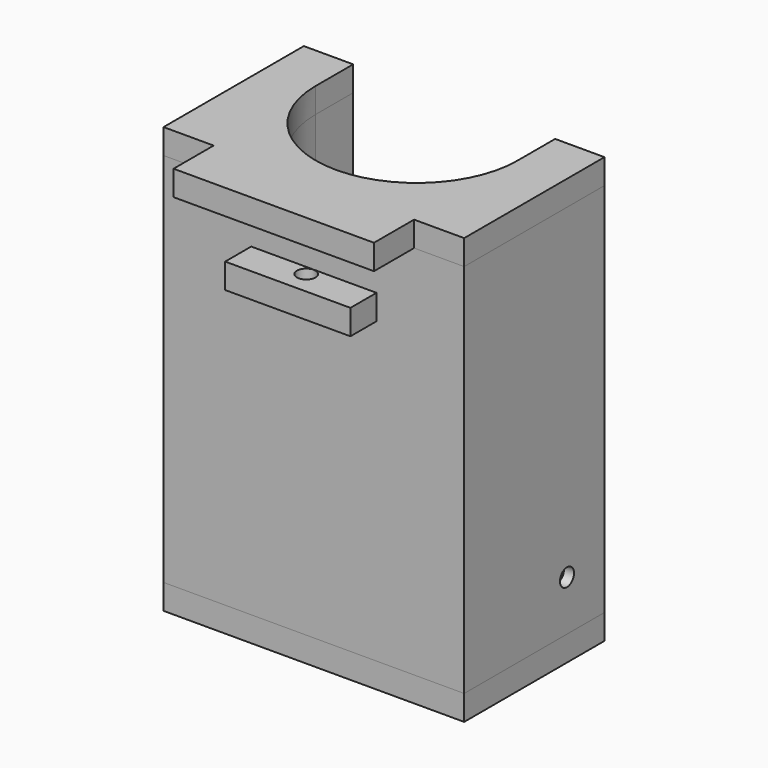
from build123d import *

# Parameters (mm, degrees)
F1_DEPTH  = 5
F3_DEPTH  = 2.1
F5_DEPTH  = 8.2
F7_DEPTH  = 60
F10_DEPTH = 5
F12_W     = 25
F12_H     = 6.5
F12_R     = 1.85
F13_DEPTH = 5
F15_R     = 1.75
F16_DEPTH = 3
F17_R     = 1.75
F18_DEPTH = 10
F20_W     = 3
F20_H     = 6.2998386914
F21_DEPTH = 25


# Not quite as in the source:
# - a pattern or mirror of a feature is missing from the dataset's text; its kind, count and spacing are read off the source's solid
# - a feature names something its author has since deleted; it is built from what else it names


with BuildPart() as f1:
    # F0 (on Top) → F1 (new body)
    with BuildSketch(Plane.XY):
        with BuildLine():
            Line((-20.15, 24), (-30, 24))
            Line((-30, 24), (-30, -11))
            Line((-30, -11), (-12.5, -11))
            Line((-12.5, -11), (30, -11))
            Line((30, -11), (30, 24))
            Line((30, 24), (20.15, 24))
            Line((20.15, 24), (20.15, 14.65))
            ThreePointArc((20.15, 14.65), (0, -5.5), (-20.15, 14.65))
            Line((-20.15, 14.65), (-20.15, 24))
        make_face()
    extrude(amount=F1_DEPTH)

    # F2 (on face) → F3 (join)
    with BuildSketch(Plane.XY.offset(5)):
        with BuildLine():
            Line((-20.15, 24), (-30, 24))
            Line((-30, 24), (-30, -11))
            Line((-30, -11), (30, -11))
            Line((30, -11), (30, 24))
            Line((30, 24), (20.15, 24))
            Line((20.15, 24), (20.15, 14.65))
            ThreePointArc((20.15, 14.65), (0, -5.5), (-20.15, 14.65))
            Line((-20.15, 14.65), (-20.15, 24))
        make_face()
    extrude(amount=F3_DEPTH)

    # F4 (on face) → F5 (join)
    with BuildSketch(Plane.XY.offset(7.1)):
        with BuildLine():
            Line((-22.6, 24), (-30, 24))
            Line((-30, 24), (-30, -11))
            Line((-30, -11), (30, -11))
            Line((30, -11), (30, 24))
            Line((30, 24), (22.6, 24))
            Line((22.6, 24), (22.6, 14.65))
            ThreePointArc((22.6, 14.65), (0, -7.95), (-22.6, 14.65))
            Line((-22.6, 14.65), (-22.6, 24))
        make_face()
    extrude(amount=F5_DEPTH)

    # F6 (on face) → F7 (join)
    with BuildSketch(Plane.XY.offset(15.3)):
        with BuildLine():
            Line((-20.15, 24), (-30, 24))
            Line((-30, 24), (-30, -11))
            Line((-30, -11), (30, -11))
            Line((30, -11), (30, 24))
            Line((30, 24), (20.15, 24))
            Line((20.15, 24), (20.15, 14.65))
            ThreePointArc((20.15, 14.65), (0, -5.5), (-20.15, 14.65))
            Line((-20.15, 14.65), (-20.15, 24))
        make_face()
    extrude(amount=F7_DEPTH)

    # F12 (on offset) → F13 (join)
    with BuildSketch(Plane.XY.offset(64.7)):
        with Locations((0, -14.25)):
            Rectangle(F12_W, F12_H)
        with Locations((0, -12.9)):
            Circle(F12_R, mode=Mode.SUBTRACT)
    extrude(amount=-F13_DEPTH)

    # F15 (on offset) → F16 (cut)
    with BuildSketch(Plane.YZ.offset(25)):
        Polygon((11.0127864357, 10.0260285901), (12.8088517975, 6.8630949494), (16.4460653619, 6.8370663592), (18.2872135643, 9.9739714099), (16.4911482025, 13.1369050506), (12.8539346381, 13.1629336408), align=None)
        with Locations((14.65, 10)):
            Circle(F15_R, mode=Mode.SUBTRACT)
    f16 = extrude(amount=F16_DEPTH, mode=Mode.SUBTRACT)

    # F16_copies: F16 across plane
    add(f16.mirror(Plane(origin=(0, 0, 0), x_dir=(0, 0, -1), z_dir=(-1, 0, 0))), mode=Mode.SUBTRACT)

    # F17 (on face) → F18 (cut)
    with BuildSketch(Plane.YZ.offset(30)):
        with Locations((14.65, 10)):
            Circle(F17_R)
    f18 = extrude(amount=-F18_DEPTH, mode=Mode.SUBTRACT)

    # F18_copies: F18 across plane
    add(f18.mirror(Plane(origin=(0, 0, 0), x_dir=(0, 0, -1), z_dir=(-1, 0, 0))), mode=Mode.SUBTRACT)

    # F20 (on plane+point) → F21 (cut)
    with BuildSketch(Plane.XZ.offset(-11.0127864357)):
        with Locations((26.5, 10.0130142951)):
            Rectangle(F20_W, F20_H)
    f21 = extrude(amount=-F21_DEPTH, mode=Mode.SUBTRACT)

    # F21_copies: F21 across plane
    add(f21.mirror(Plane(origin=(0, 0, 0), x_dir=(0, 0, -1), z_dir=(-1, 0, 0))), mode=Mode.SUBTRACT)


with BuildPart() as f10:
    # F9 (on offset) → F10 (new body)
    with BuildSketch(Plane.XY.offset(80)):
        with BuildLine():
            Line((-20.15, 24), (-30, 24))
            Line((-30, 24), (-30, -11))
            Line((-30, -11), (-20, -11))
            Line((-20, -11), (-20, -21))
            Line((-20, -21), (20, -21))
            Line((20, -21), (20, -11))
            Line((20, -11), (30, -11))
            Line((30, -11), (30, 24))
            Line((30, 24), (20.15, 24))
            Line((20.15, 24), (20.15, 14.65))
            ThreePointArc((20.15, 14.65), (0, -5.5), (-20.15, 14.65))
            Line((-20.15, 14.65), (-20.15, 24))
        make_face()
    extrude(amount=-F10_DEPTH)


with BuildPart() as f10b:
    # F0 (on Top) → F10, piece 2 (new body)
    with BuildSketch(Plane.XY):
        with BuildLine():
            Line((-20.15, 24), (-30, 24))
            Line((-30, 24), (-30, -11))
            Line((-30, -11), (-12.5, -11))
            Line((-12.5, -11), (30, -11))
            Line((30, -11), (30, 24))
            Line((30, 24), (20.15, 24))
            Line((20.15, 24), (20.15, 14.65))
            ThreePointArc((20.15, 14.65), (0, -5.5), (-20.15, 14.65))
            Line((-20.15, 14.65), (-20.15, 24))
        make_face()
    extrude(amount=-F10_DEPTH)


solid = Compound([f1.part, f10.part, f10b.part])
